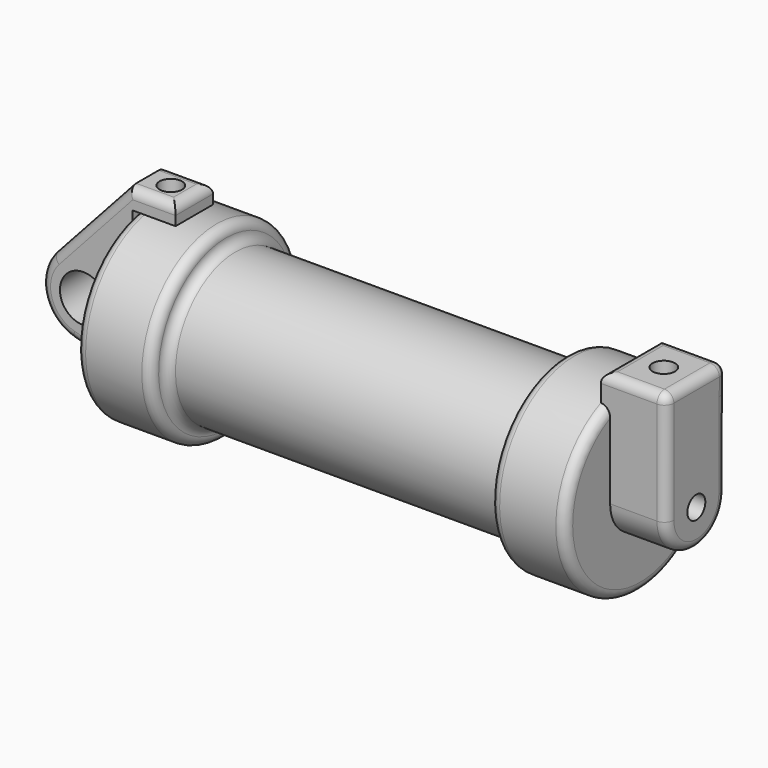
from build123d import *

# Parameters (mm, degrees)
F0_W          = 5.842
F0_H          = 12.7
F0_R          = 3.175
F2_DEPTH      = 3.175
F3_R          = 1.524
F4_DEPTH      = 7.62
F4_DEPTH_BACK = 1.27
F5_R          = 1.524
F6_DEPTH      = 17.78
F7_R          = 1.524
F8_DEPTH      = 10.414
F9_R          = 1.26999
F9_2_R        = 1.26999


# Not quite as in the source:
# - a fillet or chamfer is up to 0.001 mm smaller than in the source, because OpenCascade refuses the exact size
# - ends of sketch curves that miss each other by under 0.0002 mm in the source are joined


with BuildPart() as f1:
    # F0 (on Front) → F1 (revolve)
    with BuildSketch(Plane.XZ):
        Polygon((5.842, 12.7), (5.842, 0), (66.294, 0), (66.294, 12.7), (56.134, 12.7), (56.134, 10.16), (10.16, 10.16), (10.16, 12.7), align=None)
        with Locations((2.921, 6.35)):
            Rectangle(F0_W, F0_H)
    revolve(axis=Axis((33.147, 0, 0), (-1, 0, 0)))

    # F3 (on face) → F4 (join, two sides)
    with BuildSketch(Plane.YZ.offset(66.294)) as f4_sk:
        with BuildLine():
            ThreePointArc((-5.08, 0), (0, 5.08), (5.08, 0))
            Line((5.08, 0), (5.1504032361, 11.6087616267))
            ThreePointArc((5.1504032361, 11.6087616267), (0.0384591199, 12.6999417674), (-5.08, 11.6397422652))
            Line((-5.08, 11.6397422652), (-5.08, 0))
        make_face()
        with BuildLine():
            ThreePointArc((5.0799068281, -0.0307671549), (5.079976707, -0.015383648), (5.08, 0))
            ThreePointArc((5.08, 0), (0, 5.08), (-5.08, 0))
            ThreePointArc((-5.08, 0), (-0.015383648, -5.079976707), (5.0799068281, -0.0307671549))
        make_face()
        Circle(F3_R, mode=Mode.SUBTRACT)
        with BuildLine():
            ThreePointArc((-5.08, 11.6397422652), (0.0384591199, 12.6999417674), (5.1504032361, 11.6087616267))
            Line((5.1504032361, 11.6087616267), (5.1723960715, 15.2399571309))
            Line((5.1723960715, 15.2399571309), (-5.08, 15.2399571309))
            Line((-5.08, 15.2399571309), (-5.08, 11.6397422652))
        make_face()
    extrude(amount=F4_DEPTH)
    extrude(f4_sk.sketch, amount=-F4_DEPTH_BACK)

    # F7 (on face) → F8 (cut)
    with BuildSketch(Plane.XY.offset(15.2399571309)):
        with Locations((69.469, 0.0461980357)):
            Circle(F7_R)
    extrude(amount=-F8_DEPTH, mode=Mode.SUBTRACT)

    # F9 (radius 1.27 in the source; OpenCascade refuses exactly that, so slightly less here)
    f9_edges = [f1.edges().sort_by_distance(p)[0] for p in [
        (66.294, -0.038459, -12.699942),
        (10.16, 0, -12.7),
        (0, 0, -12.7),
        (69.469, 5.172396, 15.239957),
        (73.914, 0, -5.08),
        (73.914, 0.046198, 15.239957),
        (69.469, -5.08, 15.239957),
        (65.024, 0.046198, 15.239957),
        (10.16, 0, -10.16),
        (56.134, 0, -12.7),
        (73.914, -5.08, 7.619979),
        (73.914, 5.115202, 5.804381),
    ]]
    fillet(f9_edges, radius=F9_R)


with BuildPart() as f2:
    # F0 (on Front) → F2 (new body, symmetric)
    with BuildSketch(Plane.XZ):
        with BuildLine():
            Line((5.842, 0), (0, 0))
            Line((0, 0), (-0.9398, 0))
            ThreePointArc((-0.9398, 0), (-3.1957909266, -4.5493385486), (-8.1826630726, -5.5069827884))
            Line((-8.1826630726, -5.5069827884), (5.842, -9.398))
            Line((5.842, -9.398), (5.842, 0))
        make_face()
        with BuildLine():
            ThreePointArc((-8.1826630726, -5.5069827884), (-3.1957909266, -4.5493385486), (-0.9398, 0))
            ThreePointArc((-0.9398, 0), (-4.5919612295, 5.3297205562), (-10.8806298187, 3.8475430269))
            ThreePointArc((-10.8806298187, 3.8475430269), (-12.1459778134, -1.5837270034), (-8.1826630726, -5.5069827884))
        make_face()
        with Locations((-6.6548, 0)):
            Circle(F0_R, mode=Mode.SUBTRACT)
        with BuildLine():
            Line((-0.9398, 0), (0, 0))
            Line((0, 0), (0, 12.7))
            Line((0, 12.7), (5.842, 12.7))
            Line((5.842, 12.7), (5.842, 15.24))
            Line((5.842, 15.24), (-0.508, 15.24))
            Line((-0.508, 15.24), (-10.8806298187, 3.8475430269))
            ThreePointArc((-10.8806298187, 3.8475430269), (-4.5919612295, 5.3297205562), (-0.9398, 0))
        make_face()
    extrude(amount=F2_DEPTH, both=True)

    # F5 (on face) → F6 (cut)
    with BuildSketch(Plane.XY.offset(15.24)):
        with Locations((2.667, 0)):
            Circle(F5_R)
    extrude(amount=-F6_DEPTH, mode=Mode.SUBTRACT)

    # F9#2 (radius 1.27 in the source; OpenCascade refuses exactly that, so slightly less here)
    f9_2_edges = [f2.edges().sort_by_distance(p)[0] for p in [
        (5.842, 0, 15.24),
        (2.667, 3.175, 15.24),
        (-5.694315, 3.175, 9.543772),
        (-12.145978, 3.175, -1.583727),
        (-5.694315, -3.175, 9.543772),
        (-12.145978, -3.175, -1.583727),
        (-1.170332, -3.175, -7.452491),
        (-1.170332, 3.175, -7.452491),
        (5.842, 0, -9.398),
        (-8.182663, 0, -5.506983),
        (2.667, -3.175, 15.24),
    ]]
    fillet(f9_2_edges, radius=F9_2_R)


solid = Compound([f1.part, f2.part])
